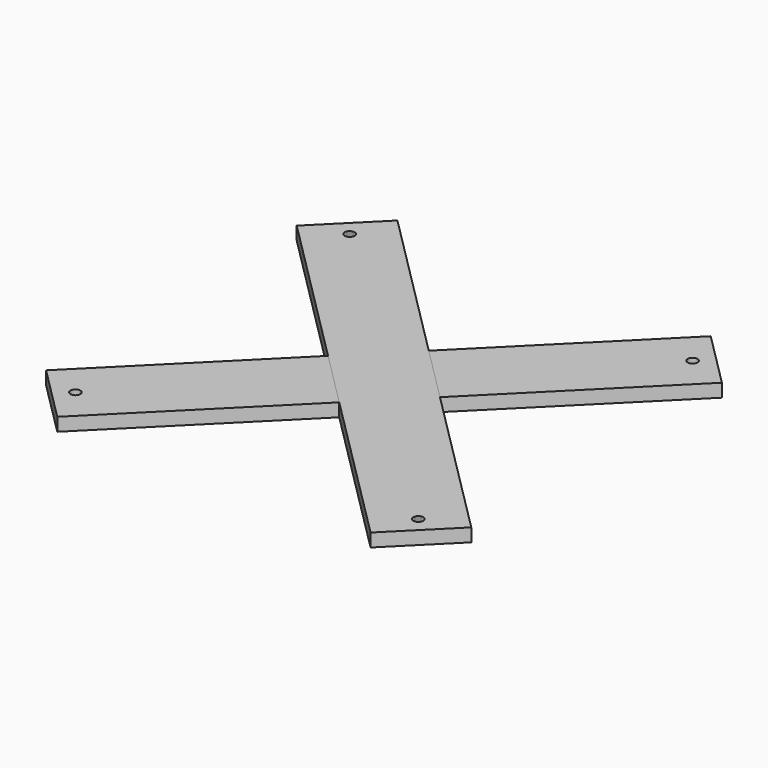
from build123d import *

# Parameters (mm, degrees)
F1_E1_W       = 251.4471713899
F1_E1_H       = 6.35
F2_DEPTH      = 19.05
F2_DEPTH_BACK = 19.05
F3_D          = 4.7625
F5_COUNT      = 2
F5_ANGLE      = 90


with BuildPart() as f2:
    # F1_E1 (on explicit) → F2 (new body, two sides)
    with BuildSketch(Plane(origin=(-88.9, -88.9, 0), x_dir=(0.7071067812, 0.7071067812, 0), z_dir=(-0.7071067812, 0.7071067812, 0))) as f2_sk:
        with Locations((125.723585695, 3.175)):
            Rectangle(F1_E1_W, F1_E1_H)
    extrude(amount=F2_DEPTH)
    extrude(f2_sk.sketch, amount=-F2_DEPTH_BACK)

    # F3 (through all)
    with Locations(Plane.XY):
        with Locations((-82.55, -82.55), (82.55, 82.55)):
            Hole(F3_D / 2)


with BuildPart() as f5_1:
    # F5: instance of F2
    add(f2.part.rotate(Axis((0, 0, 23.5672015697), (0, 0, 1)), 1 * F5_ANGLE / (F5_COUNT - 1)))


with BuildPart() as f5_2:
    # F5: instance of F2
    add(f2.part.rotate(Axis((0, 0, 23.5672015697), (0, 0, 1)), -1 * F5_ANGLE / (F5_COUNT - 1)))


solid = Compound([f2.part, f5_1.part, f5_2.part])
